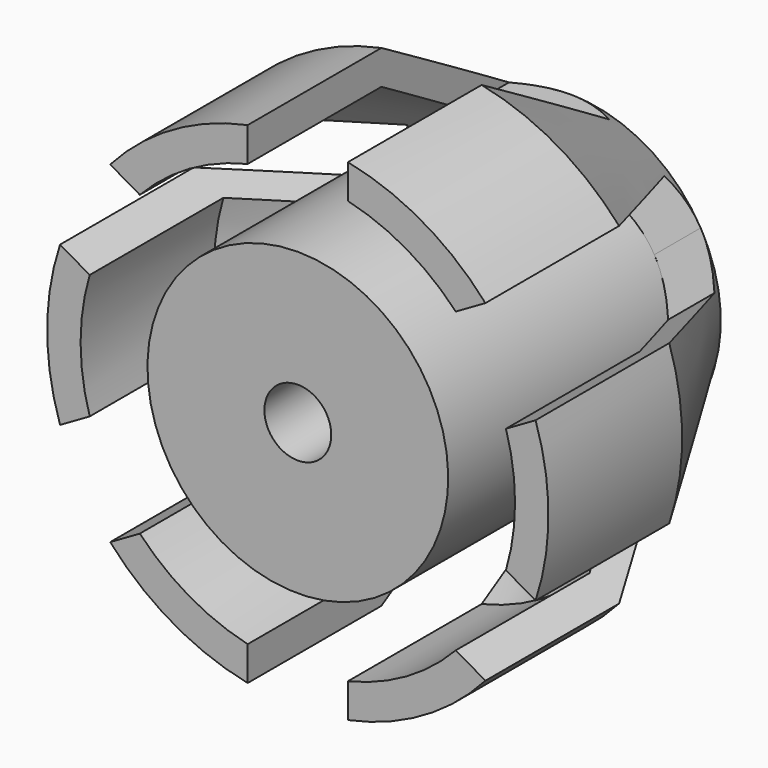
from build123d import *

# Parameters (mm, degrees)
F3_DEPTH = 25
F4_R     = 3
F5_DEPTH = 7
F6_R     = 1
F7_DEPTH = 25


# Not quite as in the source:
# - a feature names something its author has since deleted; it is built from what else it names


with BuildPart() as f1:
    # F0 (on Right) → F1 (revolve)
    with BuildSketch(Plane.YZ):
        Polygon((6.6886462844, 0), (16.8847987071, 0), (16.8847987071, 4.5), (11.6886462844, 7.5), (6.6886462844, 7.5), (6.6886462844, 6.5), (11.6886462844, 6.5), (15.1527478995, 4.5), (6.6886462844, 4.5), align=None)
    revolve(axis=Axis((0, 8.4423993535, 0), (0, 1, 0)))

    # F2 (on face) → F3 (cut)
    with BuildSketch(Plane(origin=(0, 16.8847987071, 0), x_dir=(-1, 0, 0), z_dir=(0, 1, 0))):
        with BuildLine():
            ThreePointArc((-7.1139610307, -2.3751965085), (-6.4951905284, -3.75), (-5.6139610307, -4.9732727199))
            Line((-5.6139610307, -4.9732727199), (-3.147114317, -3.5490381057))
            Line((-3.147114317, -3.5490381057), (-3.8971148018, -2.2499991604))
            Line((-3.8971148018, -2.2499991604), (-4.647114317, -0.9509618943))
            Line((-4.647114317, -0.9509618943), (-7.1139610307, -2.3751965085))
        make_face()
        with BuildLine():
            Line((-3.147114317, 3.5490381057), (-5.6139610307, 4.9732727199))
            ThreePointArc((-5.6139610307, 4.9732727199), (-6.4951905284, 3.75), (-7.1139610307, 2.3751965085))
            Line((-7.1139610307, 2.3751965085), (-4.647114317, 0.9509618943))
            Line((-4.647114317, 0.9509618943), (-3.8971148073, 2.2499991508))
            Line((-3.8971148073, 2.2499991508), (-3.147114317, 3.5490381057))
        make_face()
        with BuildLine():
            Line((1.5, 4.5), (1.5, 7.3484692283))
            ThreePointArc((1.5, 7.3484692283), (0, 7.5), (-1.5, 7.3484692283))
            Line((-1.5, 7.3484692283), (-1.5, 4.5))
            Line((-1.5, 4.5), (0, 4.5))
            Line((0, 4.5), (1.5, 4.5))
        make_face()
        with BuildLine():
            Line((4.647114317, 0.9509618943), (7.1139610307, 2.3751965085))
            ThreePointArc((7.1139610307, 2.3751965085), (6.4951905284, 3.75), (5.6139610307, 4.9732727199))
            Line((5.6139610307, 4.9732727199), (3.147114317, 3.5490381057))
            Line((3.147114317, 3.5490381057), (3.8971147984, 2.2499991663))
            Line((3.8971147984, 2.2499991663), (4.647114317, 0.9509618943))
        make_face()
        with BuildLine():
            ThreePointArc((5.6139610307, -4.9732727199), (6.4951905284, -3.75), (7.1139610307, -2.3751965085))
            Line((7.1139610307, -2.3751965085), (4.647114317, -0.9509618943))
            Line((4.647114317, -0.9509618943), (3.8971147929, -2.2499991758))
            Line((3.8971147929, -2.2499991758), (3.147114317, -3.5490381057))
            Line((3.147114317, -3.5490381057), (5.6139610307, -4.9732727199))
        make_face()
        with BuildLine():
            ThreePointArc((-1.5, -7.3484692283), (0, -7.5), (1.5, -7.3484692283))
            Line((1.5, -7.3484692283), (1.5, -4.5))
            Line((1.5, -4.5), (0, -4.5))
            Line((0, -4.5), (-1.5, -4.5))
            Line((-1.5, -4.5), (-1.5, -7.3484692283))
        make_face()
    extrude(amount=-F3_DEPTH, mode=Mode.SUBTRACT)

    # F4 (on face) → F5 (cut)
    with BuildSketch(Plane(origin=(0, 16.8847987071, 0), x_dir=(-1, 0, 0), z_dir=(0, 1, 0))):
        Circle(F4_R)
    extrude(amount=-F5_DEPTH, mode=Mode.SUBTRACT)

    # F6 (on face) → F7 (cut)
    with BuildSketch(Plane(origin=(0, 9.8847987071, 0), x_dir=(-1, 0, 0), z_dir=(0, 1, 0))):
        Circle(F6_R)
    extrude(amount=-F7_DEPTH, mode=Mode.SUBTRACT)


solid = f1.part
